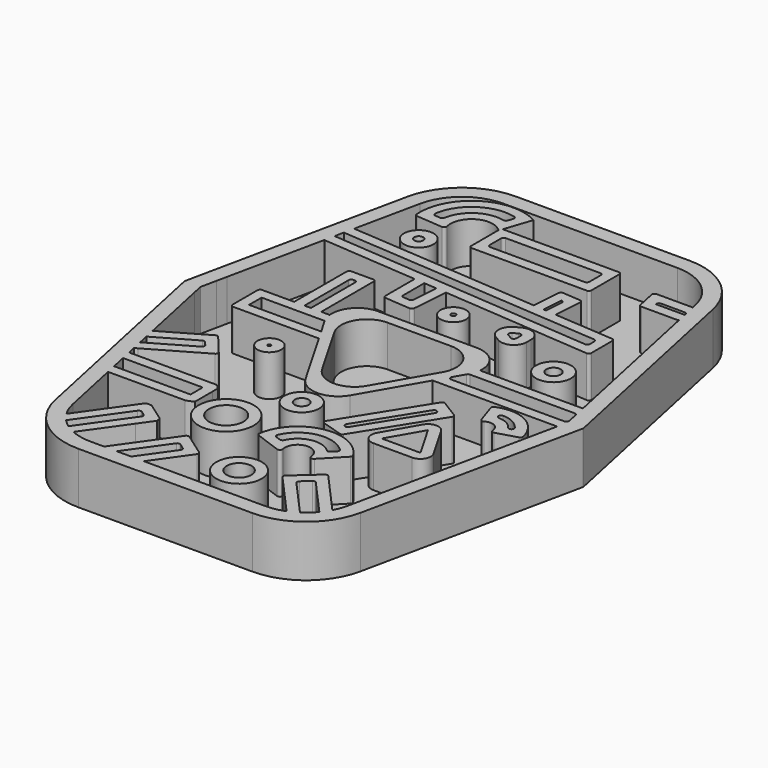
from build123d import *

# Parameters (mm, degrees)
F1_DEPTH = 10
F0_R     = 3.399072215
F0_R_2   = 1.3990718871
F0_R_3   = 2.4667891004
F0_R_4   = 0.4667891482
F0_R_5   = 2.8692483902
F0_R_6   = 0.8692480624
F0_R_7   = 2.3127347231
F0_R_8   = 0.3127347231
F0_R_9   = 4.3970015831
F0_R_10  = 2.39700148
F0_R_11  = 5.3427862003
F0_R_12  = 3.3427864912
F0_R_13  = 3.3629990648
F0_R_14  = 1.3629989638
F2_DEPTH = 2


with BuildPart() as f1:
    # F0 (on Top) → F1 (new body)
    with BuildSketch(Plane.XY):
        with BuildLine():
            ThreePointArc((-38.6444153976, 0.1036928032), (-38.6525607435, 0.0521305146), (-38.6552857598, 0))
            ThreePointArc((-38.6552857598, 0), (-38.6525607435, -0.0521305146), (-38.6444153976, -0.1036928032))
            Line((-38.6444153976, -0.1036928032), (-29.6150769124, -42.6960128826))
            ThreePointArc((-29.6150769124, -42.6960128826), (-25.081587821, -50.1006971906), (-16.8977063297, -53))
            Line((-16.8977063297, -53), (0, -53))
            Line((0, -53), (16.8977063297, -53))
            ThreePointArc((16.8977063297, -53), (25.081587821, -50.1006971906), (29.6150769124, -42.6960128826))
            Line((29.6150769124, -42.6960128826), (38.6444153976, -0.1036928032))
            ThreePointArc((38.6444153976, -0.1036928032), (38.6552857598, 0), (38.6444153976, 0.1036928032))
            Line((38.6444153976, 0.1036928032), (29.6150769124, 42.6960128826))
            ThreePointArc((29.6150769124, 42.6960128826), (25.081587821, 50.1006971906), (16.8977063297, 53))
            Line((16.8977063297, 53), (0, 53))
            Line((0, 53), (-16.8977063297, 53))
            ThreePointArc((-16.8977063297, 53), (-25.081587821, 50.1006971906), (-29.6150769124, 42.6960128826))
            Line((-29.6150769124, 42.6960128826), (-38.6444153976, 0.1036928032))
        make_face()
        with BuildLine():
            Line((-16.8977063297, -40), (-22.671018251, -48.1651007012))
            ThreePointArc((-22.671018251, -48.1651007012), (-23.462448413, -47.5434846975), (-24.1873929575, -46.8454706828))
            Line((-24.1873929575, -46.8454706828), (-17.6647293923, -37.6205741976))
            ThreePointArc((-17.6647293923, -37.6205741976), (-17.3410368605, -37.4164424895), (-16.9678087612, -37.5009847586))
            Line((-16.9678087612, -37.5009847586), (-16.1512996793, -38.078315252))
            ThreePointArc((-16.1512996793, -38.078315252), (-15.9471679712, -38.4020077838), (-16.0317102403, -38.7752358831))
            Line((-16.0317102403, -38.7752358831), (-16.8977063297, -40))
        make_face(mode=Mode.SUBTRACT)
        Polygon((-14.7321429104, -28.4901845949), (-29.5599630094, -28.4901845949), (-30.1859044805, -25.5375541747), (-14.7321429104, -25.5375541747), align=None, mode=Mode.SUBTRACT)
        with BuildLine():
            Line((-9.03667927, -50), (-11.8329823017, -50))
            Line((-11.8329823017, -50), (-6.4127478404, -42.3342509803))
            ThreePointArc((-6.4127478404, -42.3342509803), (-6.0890553086, -42.1301192721), (-5.7158272093, -42.2146615413))
            Line((-5.7158272093, -42.2146615413), (-4.6680736615, -42.9554984604))
            ThreePointArc((-4.6680736615, -42.9554984604), (-4.4639419533, -43.2791909922), (-4.5484842225, -43.6524190915))
            Line((-4.5484842225, -43.6524190915), (-9.03667927, -50))
        make_face(mode=Mode.SUBTRACT)
        with BuildLine():
            Line((-23.2424551979, -15.1969495596), (-31.3818357551, -19.8962231153))
            Line((-31.3818357551, -19.8962231153), (-31.8192990802, -17.8326635315))
            Line((-31.8192990802, -17.8326635315), (-24.3936597276, -13.5454686523))
            ThreePointArc((-24.3936597276, -13.5454686523), (-24.05538108, -13.486336172), (-23.758744916, -13.6593566327))
            Line((-23.758744916, -13.6593566327), (-23.1075403864, -14.4448121362))
            ThreePointArc((-23.1075403864, -14.4448121362), (-23.0003100157, -14.8522155052), (-23.2424551979, -15.1969495596))
        make_face(mode=Mode.SUBTRACT)
        with BuildLine():
            ThreePointArc((24.5828640799, -46.3983083979), (23.5576252344, -47.4595898133), (22.3873711213, -48.3584436635))
            Line((22.3873711213, -48.3584436635), (15.9027415925, -41.1162009459))
            ThreePointArc((15.9027415925, -41.1162009459), (15.7760011816, -40.7551144222), (15.9417089072, -40.4101686886))
            Line((15.9417089072, -40.4101686886), (17.3893763061, -39.1139422117))
            ThreePointArc((17.3893763061, -39.1139422117), (17.7504628298, -38.9872018008), (18.0954085634, -39.1529095263))
            Line((18.0954085634, -39.1529095263), (24.5828640799, -46.3983083979))
        make_face(mode=Mode.SUBTRACT)
        with BuildLine():
            ThreePointArc((-10.4824310448, 1.0520343855), (-10.4824310448, 6.0520343855), (-6.1523040259, 8.5520343855))
            Line((-6.1523040259, 8.5520343855), (6.1523040259, 8.5520343855))
            ThreePointArc((6.1523040259, 8.5520343855), (10.4824310448, 6.0520343855), (10.4824310448, 1.0520343855))
            Line((10.4824310448, 1.0520343855), (9.8750387092, 0))
            Line((9.8750387092, 0), (8.720338116, -2.000000095))
            Line((8.720338116, -2.000000095), (4.3301270189, -9.604068771))
            ThreePointArc((4.3301270189, -9.604068771), (0, -12.104068771), (-4.3301270189, -9.604068771))
            Line((-4.3301270189, -9.604068771), (-8.720338116, -2.000000095))
            Line((-8.720338116, -2.000000095), (-9.8750387092, 0))
            Line((-9.8750387092, 0), (-10.4824310448, 1.0520343855))
        make_face(mode=Mode.SUBTRACT)
        Polygon((-12.1844401645, 0), (-26.1760037392, 0), (-26.1760037392, 3.0520347133), (-13.9465332278, 3.0520347133), align=None, mode=Mode.SUBTRACT)
        with BuildLine():
            Line((-18.213680014, 15.7631627172), (-18.213680014, 5.0520347431))
            Line((-18.213680014, 5.0520347431), (-19.4621123374, 5.0520347431))
            Line((-19.4621123374, 5.0520347431), (-19.4621123374, 15.7631627172))
            ThreePointArc((-19.4621123374, 15.7631627172), (-19.3156657279, 16.1167161078), (-18.9621123374, 16.2631627172))
            Line((-18.9621123374, 16.2631627172), (-18.713680014, 16.2631627172))
            ThreePointArc((-18.713680014, 16.2631627172), (-18.3601266234, 16.1167161078), (-18.213680014, 15.7631627172))
        make_face(mode=Mode.SUBTRACT)
        with BuildLine():
            Line((9.6164062089, 10.5520347133), (-9.6164062089, 10.5520347133))
            ThreePointArc((-9.6164062089, 10.5520347133), (-13.3245054424, 8.9061366907), (-14.5913433974, 5.0520347431))
            Line((-14.5913433974, 5.0520347431), (-16.2136796862, 5.0520347431))
            Line((-16.2136796862, 5.0520347431), (-16.2136796862, 17.763163045))
            ThreePointArc((-16.2136796862, 17.763163045), (-16.3601262956, 18.1167164356), (-16.7136796862, 18.263163045))
            Line((-16.7136796862, 18.263163045), (-20.9621126652, 18.263163045))
            ThreePointArc((-20.9621126652, 18.263163045), (-21.3156660558, 18.1167164356), (-21.4621126652, 17.763163045))
            Line((-21.4621126652, 17.763163045), (-21.4621126652, 5.0520347431))
            Line((-21.4621126652, 5.0520347431), (-27.6760040671, 5.0520347431))
            ThreePointArc((-27.6760040671, 5.0520347431), (-28.0295574577, 4.9055881337), (-28.1760040671, 4.5520347431))
            Line((-28.1760040671, 4.5520347431), (-28.1760040671, 0))
            Line((-28.1760040671, 0), (-28.1760040671, -1.500000095))
            ThreePointArc((-28.1760040671, -1.500000095), (-28.0295574577, -1.8535534856), (-27.6760040671, -2.000000095))
            Line((-27.6760040671, -2.000000095), (-12.1844401645, -2.000000095))
            Line((-12.1844401645, -2.000000095), (-11.0297395713, -2.000000095))
            Line((-11.0297395713, -2.000000095), (-4.3301270189, -13.6040694267))
            ThreePointArc((-4.3301270189, -13.6040694267), (0, -16.1040694267), (4.3301270189, -13.6040694267))
            Line((4.3301270189, -13.6040694267), (11.0297395713, -2.000000095))
            Line((11.0297395713, -2.000000095), (35.1757369785, -2.000000095))
            Line((35.1757369785, -2.000000095), (26.6802990856, -42.0738560635))
            ThreePointArc((26.6802990856, -42.0738560635), (26.297566954, -43.4121284038), (25.7327165891, -44.6842922322))
            Line((25.7327165891, -44.6842922322), (18.2512778003, -36.3287808889))
            ThreePointArc((18.2512778003, -36.3287808889), (17.9063320668, -36.1630731634), (17.545245543, -36.2898135743))
            Line((17.545245543, -36.2898135743), (13.1175802697, -40.2542994517))
            ThreePointArc((13.1175802697, -40.2542994517), (12.9518725442, -40.5992451852), (13.0786129551, -40.960331709))
            Line((13.0786129551, -40.960331709), (20.5530202963, -49.3079901056))
            ThreePointArc((20.5530202963, -49.3079901056), (18.7578271516, -49.8254745701), (16.8977063297, -50))
            Line((16.8977063297, -50), (0, -50))
            Line((0, -50), (-6.5872296722, -50))
            Line((-6.5872296722, -50), (-1.7608013315, -43.1740612727))
            ThreePointArc((-1.7608013315, -43.1740612727), (-1.6762590624, -42.8008331733), (-1.8803907705, -42.4771406415))
            Line((-1.8803907705, -42.4771406415), (-6.1941850281, -39.4269786503))
            ThreePointArc((-6.1941850281, -39.4269786503), (-6.5674131275, -39.3424363812), (-6.8911056593, -39.5465680893))
            Line((-6.8911056593, -39.5465680893), (-13.4660026566, -48.845337464))
            Line((-13.4660026566, -48.845337464), (-14.2824318996, -50))
            Line((-14.2824318996, -50), (-16.8977063297, -50))
            ThreePointArc((-16.8977063297, -50), (-18.9534360088, -49.7864179088), (-20.9213522792, -49.1547950973))
            Line((-20.9213522792, -49.1547950973), (-15.2646851029, -41.1546631526))
            Line((-15.2646851029, -41.1546631526), (-13.3070006372, -38.3859420058))
            ThreePointArc((-13.3070006372, -38.3859420058), (-13.374696737, -37.928816524), (-13.5192652637, -37.4899014877))
            Line((-13.5192652637, -37.4899014877), (-17.0987254889, -34.958966335))
            ThreePointArc((-17.0987254889, -34.958966335), (-17.6772138363, -34.9371997538), (-18.2537530321, -34.9894023189))
            Line((-18.2537530321, -34.9894023189), (-25.4550744561, -45.174113523))
            ThreePointArc((-25.4550744561, -45.174113523), (-26.1977837687, -43.6753992477), (-26.6802990856, -42.0738560635))
            Line((-26.6802990856, -42.0738560635), (-29.1359738983, -30.4901849227))
            Line((-29.1359738983, -30.4901849227), (-14.1564217807, -30.4901849227))
            ThreePointArc((-14.1564217807, -30.4901849227), (-13.4271673617, -30.2402174483), (-12.7321425825, -29.9066963813))
            Line((-12.7321425825, -29.9066963813), (-12.7321425825, -25.6636664271))
            Line((-12.7321425825, -25.6636664271), (-12.7558211848, -24.3296473641))
            ThreePointArc((-12.7558211848, -24.3296473641), (-13.174958101, -23.9125849047), (-13.6320888867, -23.5375538468))
            Line((-13.6320888867, -23.5375538468), (-14.7321429104, -23.5375538468))
            Line((-14.7321429104, -23.5375538468), (-30.6098935916, -23.5375538468))
            Line((-30.6098935916, -23.5375538468), (-30.9456432666, -21.9537880317))
            Line((-30.9456432666, -21.9537880317), (-30.3818358892, -21.6282736906))
            Line((-30.3818358892, -21.6282736906), (-20.1906209234, -15.7443729867))
            ThreePointArc((-20.1906209234, -15.7443729867), (-19.9484757411, -15.3996389323), (-20.0557061118, -14.9922355633))
            Line((-20.0557061118, -14.9922355633), (-23.2966388816, -11.0831588223))
            ThreePointArc((-23.2966388816, -11.0831588223), (-23.5932750456, -10.9101383616), (-23.9315536932, -10.9692708419))
            Line((-23.9315536932, -10.9692708419), (-32.2554915687, -15.7750986151))
            Line((-32.2554915687, -15.7750986151), (-35.1757369785, -2.000000095))
            Line((-35.1757369785, -2.000000095), (-35.5997260402, 0))
            Line((-35.5997260402, 0), (-34.9527114037, 3.0520347133))
            Line((-34.9527114037, 3.0520347133), (-34.5287223558, 5.0520347431))
            Line((-34.5287223558, 5.0520347431), (-30.5607553711, 23.7693438962))
            Line((-30.5607553711, 23.7693438962), (-30.3036586015, 23.7148407898))
            Line((-30.3036586015, 23.7148407898), (-11.898490251, 22.2927000705))
            Line((-11.898490251, 22.2927000705), (-11.898490251, 15.1860698793))
            ThreePointArc((-11.898490251, 15.1860698793), (-11.7654096763, 14.8464080838), (-11.4370097096, 14.6875558361))
            Line((-11.4370097096, 14.6875558361), (-6.4813007835, 14.3046353801))
            ThreePointArc((-6.4813007835, 14.3046353801), (-6.1175160348, 14.4234093925), (-5.9442672817, 14.7646299648))
            Line((-5.9442672817, 14.7646299648), (-5.4013747687, 21.7906773609))
            Line((-5.4013747687, 21.7906773609), (23.6295337142, 19.547501081))
            ThreePointArc((23.6295337142, 19.547501081), (24.0077149683, 19.679095699), (24.1680531728, 20.0460151242))
            Line((24.1680531728, 20.0460151242), (24.1680531728, 25.1655394856))
            ThreePointArc((24.1680531728, 25.1655394856), (24.0340055522, 25.5062429579), (23.7037377487, 25.664264471))
            Line((23.7037377487, 25.664264471), (12.112475713, 26.4936379369))
            Line((12.112475713, 26.4936379369), (12.5044798494, 31.972258669))
            ThreePointArc((12.5044798494, 31.972258669), (12.3836394887, 32.3353622584), (12.0414394399, 32.5066682302))
            Line((12.0414394399, 32.5066682302), (8.5309401818, 32.7578501057))
            ThreePointArc((8.5309401818, 32.7578501057), (8.1678365924, 32.637009745), (7.9965306205, 32.2948096962))
            Line((7.9965306205, 32.2948096962), (7.6045264841, 26.8161889641))
            Line((7.6045264841, 26.8161889641), (-29.3542301857, 29.4606475244))
            Line((-29.3542301857, 29.4606475244), (-26.6802990856, 42.0738560635))
            ThreePointArc((-26.6802990856, 42.0738560635), (-23.1929997846, 47.7697670697), (-16.8977063297, 50))
            Line((-16.8977063297, 50), (0, 50))
            Line((0, 50), (16.8977063297, 50))
            ThreePointArc((16.8977063297, 50), (23.1929997846, 47.7697670697), (26.6802990856, 42.0738560635))
            Line((26.6802990856, 42.0738560635), (26.8416769509, 41.3126200438))
            Line((26.8416769509, 41.3126200438), (19.8224472179, 41.3126200438))
            ThreePointArc((19.8224472179, 41.3126200438), (19.4339588644, 41.1273847165), (19.3333175801, 40.7089272406))
            Line((19.3333175801, 40.7089272406), (20.1082804097, 37.053347716))
            ThreePointArc((20.1082804097, 37.053347716), (20.2826453747, 36.7685521657), (20.5974100474, 36.6570405192))
            Line((20.5974100474, 36.6570405192), (27.4046450229, 36.6570405192))
            Line((27.4046450229, 36.6570405192), (27.8103990355, 36.7430581467))
            Line((27.8103990355, 36.7430581467), (34.5287223558, 5.0520347431))
            Line((34.5287223558, 5.0520347431), (14.5913433974, 5.0520347431))
            ThreePointArc((14.5913433974, 5.0520347431), (13.3245054424, 8.9061366907), (9.6164062089, 10.5520347133))
        make_face(mode=Mode.SUBTRACT)
        with BuildLine():
            Line((-9.8984905148, 17.0374940741), (-9.8984905148, 22.1381629856))
            Line((-9.8984905148, 22.1381629856), (-7.3954306786, 21.9447551749))
            Line((-7.3954306786, 21.9447551749), (-7.7842453776, 16.9127636888))
            ThreePointArc((-7.7842453776, 16.9127636888), (-7.9574941307, 16.5715431165), (-8.3212788794, 16.4527691041))
            Line((-8.3212788794, 16.4527691041), (-9.4370099734, 16.5389800309))
            ThreePointArc((-9.4370099734, 16.5389800309), (-9.7654099401, 16.6978322786), (-9.8984905148, 17.0374940741))
        make_face(mode=Mode.SUBTRACT)
        with BuildLine():
            Line((-30.1495807781, 25.7088968219), (-29.7729517471, 27.4854947711))
            Line((-29.7729517471, 27.4854947711), (21.70373789, 23.8022547265))
            ThreePointArc((21.70373789, 23.8022547265), (22.0340056935, 23.6442332134), (22.1680533141, 23.3035297411))
            Line((22.1680533141, 23.3035297411), (22.1680533141, 22.2065136211))
            ThreePointArc((22.1680533141, 22.2065136211), (22.0077151096, 21.8395941958), (21.6295338555, 21.7079995778))
            Line((21.6295338555, 21.7079995778), (-30.1495807781, 25.7088968219))
        make_face(mode=Mode.SUBTRACT)
        with BuildLine():
            Line((12.6174528664, 0.75), (13.8021956605, 2.8020347133))
            ThreePointArc((13.8021956605, 2.8020347133), (13.9852083624, 2.9850474152), (14.2352083624, 3.0520347133))
            Line((14.2352083624, 3.0520347133), (34.5475967202, 3.0520347133))
            ThreePointArc((34.5475967202, 3.0520347133), (34.8623613929, 2.9405230668), (35.036726358, 2.6557275165))
            Line((35.036726358, 2.6557275165), (35.4717464737, 0.6036928032))
            ThreePointArc((35.4717464737, 0.6036928032), (35.3711051894, 0.1852353273), (34.9826168359, 0))
            Line((34.9826168359, 0), (13.0504655683, 0))
            ThreePointArc((13.0504655683, 0), (12.6174528664, 0.25), (12.6174528664, 0.75))
        make_face(mode=Mode.SUBTRACT)
        with BuildLine():
            Line((10.3668416044, 30.120097031), (10.1175757714, 26.6363762404))
            Line((10.1175757714, 26.6363762404), (9.5994264256, 26.6734506606))
            Line((9.5994264256, 26.6734506606), (9.8843768344, 30.6558964365))
            Line((9.8843768344, 30.6558964365), (9.9038011949, 30.6545065922))
            ThreePointArc((9.9038011949, 30.6545065922), (10.2460012437, 30.4832006204), (10.3668416044, 30.120097031))
        make_face(mode=Mode.SUBTRACT)
        with BuildLine():
            Line((22.2908854137, 39.3126189268), (26.8605515458, 39.3126189268))
            ThreePointArc((26.8605515458, 39.3126189268), (27.1753162185, 39.2011072803), (27.3496811835, 38.91631173))
            Line((27.3496811835, 38.91631173), (27.4046450229, 38.6570416361))
            Line((27.4046450229, 38.6570416361), (21.8127550029, 38.6570416361))
            Line((21.8127550029, 38.6570416361), (21.8017557759, 38.7089261237))
            ThreePointArc((21.8017557759, 38.7089261237), (21.9023970602, 39.1273835996), (22.2908854137, 39.3126189268))
        make_face(mode=Mode.SUBTRACT)
    extrude(amount=F1_DEPTH)


with BuildPart() as f1b:
    # F0 (on Top) → F1, piece 2 (new body)
    with BuildSketch(Plane.XY):
        with BuildLine():
            Line((11.3479569554, 40), (11.3479569554, 42.8686450124))
            ThreePointArc((11.3479569554, 42.8686450124), (11.201510346, 43.222198403), (10.8479569554, 43.3686450124))
            Line((10.8479569554, 43.3686450124), (-11.6518868951, 43.3686450124))
            Line((-11.6518868951, 43.3686450124), (-9.9092187502, 48.610936098))
            ThreePointArc((-9.9092187502, 48.610936098), (-20.2784683686, 48.3517526151), (-24.9408979548, 39.0862108565))
            ThreePointArc((-24.9408979548, 39.0862108565), (-24.7965040915, 38.7701226352), (-24.4809901003, 38.6244782986))
            Line((-24.4809901003, 38.6244782986), (-19.372677463, 38.2275064133))
            ThreePointArc((-19.372677463, 38.2275064133), (-18.9524686823, 38.402768931), (-18.8485632614, 38.8460476615))
            ThreePointArc((-18.8485632614, 38.8460476615), (-16.8871391154, 43.3911768549), (-11.9827720337, 42.7184454137))
            Line((-11.9827720337, 42.7184454137), (-11.9827720337, 36.1013327837))
            ThreePointArc((-11.9827720337, 36.1013327837), (-11.8363254243, 35.7477793931), (-11.4827720337, 35.6013327837))
            Line((-11.4827720337, 35.6013327837), (10.8479569554, 35.6013327837))
            ThreePointArc((10.8479569554, 35.6013327837), (11.201510346, 35.7477793931), (11.3479569554, 36.1013327837))
            Line((11.3479569554, 36.1013327837), (11.3479569554, 40))
        make_face()
        with BuildLine():
            Line((9.3479566276, 40.8686446846), (9.3479566276, 40))
            Line((9.3479566276, 40), (9.3479566276, 38.1013331115))
            ThreePointArc((9.3479566276, 38.1013331115), (9.2015100182, 37.7477797209), (8.8479566276, 37.6013331115))
            Line((8.8479566276, 37.6013331115), (-9.4827717058, 37.6013331115))
            ThreePointArc((-9.4827717058, 37.6013331115), (-9.8363250964, 37.7477797209), (-9.9827717058, 38.1013331115))
            Line((-9.9827717058, 38.1013331115), (-9.9827717058, 40.8686446846))
            ThreePointArc((-9.9827717058, 40.8686446846), (-9.8363250964, 41.2221980751), (-9.4827717058, 41.3686446846))
            Line((-9.4827717058, 41.3686446846), (8.8479566276, 41.3686446846))
            ThreePointArc((8.8479566276, 41.3686446846), (9.2015100182, 41.2221980751), (9.3479566276, 40.8686446846))
        make_face(mode=Mode.SUBTRACT)
        with BuildLine():
            ThreePointArc((-13.4505709735, 45.7493001201), (-18.2466697127, 44.9021356054), (-20.8884646153, 40.8105380538))
            ThreePointArc((-20.8884646153, 40.8105380538), (-21.07314416, 40.4979170999), (-21.4206567051, 40.3926867524))
            Line((-21.4206567051, 40.3926867524), (-22.4207461206, 40.4704046621))
            ThreePointArc((-22.4207461206, 40.4704046621), (-22.77354721, 40.6579409406), (-22.8763290658, 41.0440424228))
            ThreePointArc((-22.8763290658, 41.0440424228), (-19.3529933545, 46.5682854362), (-12.8944386724, 47.6720185674))
            ThreePointArc((-12.8944386724, 47.6720185674), (-12.578470645, 47.4274727229), (-12.5425237403, 47.0295452364))
            Line((-12.5425237403, 47.0295452364), (-12.8589549278, 46.0776575245))
            ThreePointArc((-12.8589549278, 46.0776575245), (-13.0907839452, 45.798205021), (-13.4505709735, 45.7493001201))
        make_face(mode=Mode.SUBTRACT)
    extrude(amount=F1_DEPTH)


with BuildPart() as f1c:
    # F0 (on Top) → F1, piece 3 (new body)
    with BuildSketch(Plane.XY):
        with Locations((23.5671252012, 11.6359107196)):
            Circle(F0_R)
        with Locations((23.5671252012, 11.6359107196)):
            Circle(F0_R_2, mode=Mode.SUBTRACT)
    extrude(amount=F1_DEPTH)


with BuildPart() as f1d:
    # F0 (on Top) → F1, piece 4 (new body)
    with BuildSketch(Plane.XY):
        with BuildLine():
            Line((14.2961637919, 16.6796022979), (14.313119636, 17.6879111175))
            ThreePointArc((14.313119636, 17.6879111175), (13.0996991626, 19.8736857525), (10.6000525651, 19.9157201145))
            Line((10.6000525651, 19.9157201145), (9.7183535904, 19.4262498964))
            ThreePointArc((9.7183535904, 19.4262498964), (8.4321274663, 17.2825096235), (9.6455479397, 15.0967349886))
            Line((9.6455479397, 15.0967349886), (10.5102910703, 14.577896387))
            ThreePointArc((10.5102910703, 14.577896387), (13.0099376678, 14.535862025), (14.2961637919, 16.6796022979))
        make_face()
        with BuildLine():
            ThreePointArc((10.6745288389, 16.8117272069), (10.4318447443, 17.2488821339), (10.6890899691, 17.6776301884))
            Line((10.6890899691, 17.6776301884), (11.5707889438, 18.1671004065))
            ThreePointArc((11.5707889438, 18.1671004065), (12.0707182633, 18.1586935341), (12.313402358, 17.7215386072))
            Line((12.313402358, 17.7215386072), (12.2964465139, 16.7132297875))
            ThreePointArc((12.2964465139, 16.7132297875), (12.0392012891, 16.2844817329), (11.5392719696, 16.2928886053))
            Line((11.5392719696, 16.2928886053), (10.6745288389, 16.8117272069))
        make_face(mode=Mode.SUBTRACT)
    extrude(amount=F1_DEPTH)


with BuildPart() as f1e:
    # F0 (on Top) → F1, piece 5 (new body)
    with BuildSketch(Plane.XY):
        with Locations((0, 16.813468188)):
            Circle(F0_R_3)
        with Locations((0, 16.813468188)):
            Circle(F0_R_4, mode=Mode.SUBTRACT)
    extrude(amount=F1_DEPTH)


with BuildPart() as f1f:
    # F0 (on Top) → F1, piece 6 (new body)
    with BuildSketch(Plane.XY):
        with Locations((-19.6312479675, 32.9623892903)):
            Circle(F0_R_5)
        with Locations((-19.6312479675, 32.9623892903)):
            Circle(F0_R_6, mode=Mode.SUBTRACT)
    extrude(amount=F1_DEPTH)


with BuildPart() as f1g:
    # F0 (on Top) → F1, piece 7 (new body)
    with BuildSketch(Plane.XY):
        with Locations((-15.4942134395, -8.4121655673)):
            Circle(F0_R_7)
        with Locations((-15.4942134395, -8.4121655673)):
            Circle(F0_R_8, mode=Mode.SUBTRACT)
    extrude(amount=F1_DEPTH)


with BuildPart() as f1h:
    # F0 (on Top) → F1, piece 8 (new body)
    with BuildSketch(Plane.XY):
        with BuildLine():
            ThreePointArc((16.9099035396, -29.31134498), (17.0474105448, -29.0174641157), (16.9755778926, -28.7010558209))
            ThreePointArc((16.9755778926, -28.7010558209), (8.0370288338, -24.8624119764), (1.3814706109, -31.9572263209))
            ThreePointArc((1.3814706109, -31.9572263209), (1.4476923266, -32.2852257943), (1.7059395028, -32.4980105827))
            Line((1.7059395028, -32.4980105827), (6.7058357347, -34.3116790255))
            ThreePointArc((6.7058357347, -34.3116790255), (7.2089344656, -34.2149809572), (7.3628591381, -33.7263440321))
            ThreePointArc((7.3628591381, -33.7263440321), (9.3831674608, -30.7137956444), (12.2334222709, -32.9572619412))
            ThreePointArc((12.2334222709, -32.9572619412), (12.5632782348, -33.3877886295), (13.0914250565, -33.2644228284))
            Line((13.0914250565, -33.2644228284), (16.9099035396, -29.31134498))
        make_face()
        with BuildLine():
            ThreePointArc((13.5579327139, -29.9027619507), (13.2087280029, -30.0552754711), (12.8534722744, -29.9174434304))
            ThreePointArc((12.8534722744, -29.9174434304), (8.9077745167, -28.7672002682), (5.6891479067, -31.3229844675))
            ThreePointArc((5.6891479067, -31.3229844675), (5.4279014723, -31.5785333578), (5.062574615, -31.5880843862))
            Line((5.062574615, -31.5880843862), (4.120345984, -31.2462992261))
            ThreePointArc((4.120345984, -31.2462992261), (3.8315880544, -30.9739599037), (3.832254111, -30.5770349678))
            ThreePointArc((3.832254111, -30.5770349678), (8.4869300114, -26.8117435782), (14.2383441665, -28.4744709171))
            ThreePointArc((14.2383441665, -28.4744709171), (14.3929775253, -28.8260001172), (14.2527028416, -29.18350154))
            Line((14.2527028416, -29.18350154), (13.5579327139, -29.9027619507))
        make_face(mode=Mode.SUBTRACT)
    extrude(amount=F1_DEPTH)


with BuildPart() as f1i:
    # F0 (on Top) → F1, piece 9 (new body)
    with BuildSketch(Plane.XY):
        with BuildLine():
            ThreePointArc((10.9588627462, -24.4177700551), (11.2812815043, -24.4095095453), (11.5315792264, -24.2061056565))
            Line((11.5315792264, -24.2061056565), (20.7565783394, -9.4918535856))
            ThreePointArc((20.7565783394, -9.4918535856), (20.820301645, -9.1145129574), (20.5985407094, -8.8026336588))
            Line((20.5985407094, -8.8026336588), (17.1937893426, -6.6680482115))
            ThreePointArc((17.1937893426, -6.6680482115), (16.8164487143, -6.604324906), (16.5045694158, -6.8260858415))
            Line((16.5045694158, -6.8260858415), (6.7180857243, -22.4359288517))
            ThreePointArc((6.7180857243, -22.4359288517), (6.6727194656, -22.8748510565), (6.992626801, -23.1787755471))
            Line((6.992626801, -23.1787755471), (10.9588627462, -24.4177700551))
        make_face()
        with BuildLine():
            Line((17.9996980174, -10.1240042467), (10.6561208163, -21.8373111766))
            ThreePointArc((10.6561208163, -21.8373111766), (10.4058230943, -22.0407150654), (10.0834043362, -22.0489755752))
            Line((10.0834043362, -22.0489755752), (10.0650914715, -22.0432549023))
            ThreePointArc((10.0650914715, -22.0432549023), (9.7451841361, -21.7393304116), (9.7905503948, -21.3004082068))
            Line((9.7905503948, -21.3004082068), (17.1367200769, -9.5829661635))
            ThreePointArc((17.1367200769, -9.5829661635), (17.4485993754, -9.361205228), (17.8259400037, -9.4249285335))
            Line((17.8259400037, -9.4249285335), (17.8416603874, -9.4347843199))
            ThreePointArc((17.8416603874, -9.4347843199), (18.063421323, -9.7466636185), (17.9996980174, -10.1240042467))
        make_face(mode=Mode.SUBTRACT)
    extrude(amount=F1_DEPTH)


with BuildPart() as f1j:
    # F0 (on Top) → F1, piece 10 (new body)
    with BuildSketch(Plane.XY):
        with BuildLine():
            Line((18.923042907, -14.1690840721), (15.1665538036, -20.6755140573))
            ThreePointArc((15.1665538036, -20.6755140573), (15.1665538036, -22.6755140573), (16.8986046112, -23.6755140573))
            Line((16.8986046112, -23.6755140573), (24.411582818, -23.6755140573))
            ThreePointArc((24.411582818, -23.6755140573), (26.1436336256, -22.6755140573), (26.1436336256, -20.6755140573))
            Line((26.1436336256, -20.6755140573), (22.3871445222, -14.1690840721))
            ThreePointArc((22.3871445222, -14.1690840721), (20.6550937146, -13.1690840721), (18.923042907, -14.1690840721))
        make_face()
        Polygon((20.6550937146, -15.1690840721), (24.411582818, -21.6755140573), (16.8986046112, -21.6755140573), align=None, mode=Mode.SUBTRACT)
    extrude(amount=F1_DEPTH)


with BuildPart() as f1k:
    # F0 (on Top) → F1, piece 11 (new body)
    with BuildSketch(Plane.XY):
        with BuildLine():
            ThreePointArc((32.8763900957, -8.4079776533), (33.1630589547, -8.1865017518), (33.2249246203, -7.8295658344))
            ThreePointArc((33.2249246203, -7.8295658344), (29.6755894977, -3.1174797736), (23.7793687223, -2.9274391838))
            ThreePointArc((23.7793687223, -2.9274391838), (23.5231046031, -3.1834847089), (23.5070086443, -3.545384598))
            Line((23.5070086443, -3.545384598), (24.8027076737, -7.3750600447))
            ThreePointArc((24.8027076737, -7.3750600447), (25.1102601617, -7.686430869), (25.5450522942, -7.6364696377))
            ThreePointArc((25.5450522942, -7.6364696377), (27.3723630932, -7.5554013738), (28.3578934548, -9.0962993995))
            ThreePointArc((28.3578934548, -9.0962993995), (28.5673105079, -9.480597228), (28.9989564669, -9.5528612523))
            Line((28.9989564669, -9.5528612523), (32.8763900957, -8.4079776533))
        make_face()
        with BuildLine():
            ThreePointArc((30.1779519109, -7.119379395), (29.875095979, -7.1131259252), (29.6314312689, -6.9331583438))
            ThreePointArc((29.6314312689, -6.9331583438), (28.293653655, -5.7802327337), (26.580839153, -5.3499387776))
            ThreePointArc((26.580839153, -5.3499387776), (26.2934192175, -5.2542799985), (26.1139781478, -5.0102272914))
            ThreePointArc((26.1139781478, -5.0102272914), (26.1833094189, -4.5557989091), (26.5943705728, -4.3500303314))
            ThreePointArc((26.5943705728, -4.3500303314), (28.7542989359, -4.8926484136), (30.4412906145, -6.346534239))
            ThreePointArc((30.4412906145, -6.346534239), (30.5096405755, -6.801111254), (30.1779519109, -7.119379395))
        make_face(mode=Mode.SUBTRACT)
    extrude(amount=F1_DEPTH)


with BuildPart() as f1l:
    # F0 (on Top) → F1, piece 12 (new body)
    with BuildSketch(Plane.XY):
        with Locations((6.5540773794, -43.3322489262)):
            Circle(F0_R_9)
        with Locations((6.5540773794, -43.3322489262)):
            Circle(F0_R_10, mode=Mode.SUBTRACT)
    extrude(amount=F1_DEPTH)


with BuildPart() as f1m:
    # F0 (on Top) → F1, piece 13 (new body)
    with BuildSketch(Plane.XY):
        with Locations((-6.242133677, -30.4548274726)):
            Circle(F0_R_11)
        with Locations((-6.242133677, -30.4548274726)):
            Circle(F0_R_12, mode=Mode.SUBTRACT)
    extrude(amount=F1_DEPTH)


with BuildPart() as f1n:
    # F0 (on Top) → F1, piece 14 (new body)
    with BuildSketch(Plane.XY):
        with Locations((0, -19.9465807527)):
            Circle(F0_R_13)
        with Locations((0, -19.9465807527)):
            Circle(F0_R_14, mode=Mode.SUBTRACT)
    extrude(amount=F1_DEPTH)


with BuildPart() as f2:
    # F0 (on Top) → F2 (new body)
    with BuildSketch(Plane.XY):
        with BuildLine():
            ThreePointArc((-14.5913433974, 5.0520347431), (-13.3245054424, 8.9061366907), (-9.6164062089, 10.5520347133))
            Line((-9.6164062089, 10.5520347133), (9.6164062089, 10.5520347133))
            ThreePointArc((9.6164062089, 10.5520347133), (13.3245054424, 8.9061366907), (14.5913433974, 5.0520347431))
            Line((14.5913433974, 5.0520347431), (34.5287223558, 5.0520347431))
            Line((34.5287223558, 5.0520347431), (27.8103990355, 36.7430581467))
            Line((27.8103990355, 36.7430581467), (27.4046450229, 36.6570405192))
            Line((27.4046450229, 36.6570405192), (20.5974100474, 36.6570405192))
            ThreePointArc((20.5974100474, 36.6570405192), (20.2826453747, 36.7685521657), (20.1082804097, 37.053347716))
            Line((20.1082804097, 37.053347716), (19.3333175801, 40.7089272406))
            ThreePointArc((19.3333175801, 40.7089272406), (19.4339588644, 41.1273847165), (19.8224472179, 41.3126200438))
            Line((19.8224472179, 41.3126200438), (26.8416769509, 41.3126200438))
            Line((26.8416769509, 41.3126200438), (26.6802990856, 42.0738560635))
            ThreePointArc((26.6802990856, 42.0738560635), (23.1929997846, 47.7697670697), (16.8977063297, 50))
            Line((16.8977063297, 50), (0, 50))
            Line((0, 50), (-16.8977063297, 50))
            ThreePointArc((-16.8977063297, 50), (-23.1929997846, 47.7697670697), (-26.6802990856, 42.0738560635))
            Line((-26.6802990856, 42.0738560635), (-29.3542301857, 29.4606475244))
            Line((-29.3542301857, 29.4606475244), (7.6045264841, 26.8161889641))
            Line((7.6045264841, 26.8161889641), (7.9965306205, 32.2948096962))
            ThreePointArc((7.9965306205, 32.2948096962), (8.1678365924, 32.637009745), (8.5309401818, 32.7578501057))
            Line((8.5309401818, 32.7578501057), (12.0414394399, 32.5066682302))
            ThreePointArc((12.0414394399, 32.5066682302), (12.3836394887, 32.3353622584), (12.5044798494, 31.972258669))
            Line((12.5044798494, 31.972258669), (12.112475713, 26.4936379369))
            Line((12.112475713, 26.4936379369), (23.7037377487, 25.664264471))
            ThreePointArc((23.7037377487, 25.664264471), (24.0340055522, 25.5062429579), (24.1680531728, 25.1655394856))
            Line((24.1680531728, 25.1655394856), (24.1680531728, 20.0460151242))
            ThreePointArc((24.1680531728, 20.0460151242), (24.0077149683, 19.679095699), (23.6295337142, 19.547501081))
            Line((23.6295337142, 19.547501081), (-5.4013747687, 21.7906773609))
            Line((-5.4013747687, 21.7906773609), (-5.9442672817, 14.7646299648))
            ThreePointArc((-5.9442672817, 14.7646299648), (-6.1175160348, 14.4234093925), (-6.4813007835, 14.3046353801))
            Line((-6.4813007835, 14.3046353801), (-11.4370097096, 14.6875558361))
            ThreePointArc((-11.4370097096, 14.6875558361), (-11.7654096763, 14.8464080838), (-11.898490251, 15.1860698793))
            Line((-11.898490251, 15.1860698793), (-11.898490251, 22.2927000705))
            Line((-11.898490251, 22.2927000705), (-30.3036586015, 23.7148407898))
            Line((-30.3036586015, 23.7148407898), (-30.5607553711, 23.7693438962))
            Line((-30.5607553711, 23.7693438962), (-34.5287223558, 5.0520347431))
            Line((-34.5287223558, 5.0520347431), (-34.9527114037, 3.0520347133))
            Line((-34.9527114037, 3.0520347133), (-35.5997260402, 0))
            Line((-35.5997260402, 0), (-35.1757369785, -2.000000095))
            Line((-35.1757369785, -2.000000095), (-32.2554915687, -15.7750986151))
            Line((-32.2554915687, -15.7750986151), (-23.9315536932, -10.9692708419))
            ThreePointArc((-23.9315536932, -10.9692708419), (-23.5932750456, -10.9101383616), (-23.2966388816, -11.0831588223))
            Line((-23.2966388816, -11.0831588223), (-20.0557061118, -14.9922355633))
            ThreePointArc((-20.0557061118, -14.9922355633), (-19.9484757411, -15.3996389323), (-20.1906209234, -15.7443729867))
            Line((-20.1906209234, -15.7443729867), (-30.3818358892, -21.6282736906))
            Line((-30.3818358892, -21.6282736906), (-30.9456432666, -21.9537880317))
            Line((-30.9456432666, -21.9537880317), (-30.6098935916, -23.5375538468))
            Line((-30.6098935916, -23.5375538468), (-14.7321429104, -23.5375538468))
            Line((-14.7321429104, -23.5375538468), (-13.6320888867, -23.5375538468))
            ThreePointArc((-13.6320888867, -23.5375538468), (-13.174958101, -23.9125849047), (-12.7558211848, -24.3296473641))
            Line((-12.7558211848, -24.3296473641), (-12.7321425825, -25.6636664271))
            Line((-12.7321425825, -25.6636664271), (-12.7321425825, -29.9066963813))
            ThreePointArc((-12.7321425825, -29.9066963813), (-13.4271673617, -30.2402174483), (-14.1564217807, -30.4901849227))
            Line((-14.1564217807, -30.4901849227), (-29.1359738983, -30.4901849227))
            Line((-29.1359738983, -30.4901849227), (-26.6802990856, -42.0738560635))
            ThreePointArc((-26.6802990856, -42.0738560635), (-26.1977837687, -43.6753992477), (-25.4550744561, -45.174113523))
            Line((-25.4550744561, -45.174113523), (-18.2537530321, -34.9894023189))
            ThreePointArc((-18.2537530321, -34.9894023189), (-17.6772138363, -34.9371997538), (-17.0987254889, -34.958966335))
            Line((-17.0987254889, -34.958966335), (-13.5192652637, -37.4899014877))
            ThreePointArc((-13.5192652637, -37.4899014877), (-13.374696737, -37.928816524), (-13.3070006372, -38.3859420058))
            Line((-13.3070006372, -38.3859420058), (-15.2646851029, -41.1546631526))
            Line((-15.2646851029, -41.1546631526), (-20.9213522792, -49.1547950973))
            ThreePointArc((-20.9213522792, -49.1547950973), (-18.9534360088, -49.7864179088), (-16.8977063297, -50))
            Line((-16.8977063297, -50), (-14.2824318996, -50))
            Line((-14.2824318996, -50), (-13.4660026566, -48.845337464))
            Line((-13.4660026566, -48.845337464), (-6.8911056593, -39.5465680893))
            ThreePointArc((-6.8911056593, -39.5465680893), (-6.5674131275, -39.3424363812), (-6.1941850281, -39.4269786503))
            Line((-6.1941850281, -39.4269786503), (-1.8803907705, -42.4771406415))
            ThreePointArc((-1.8803907705, -42.4771406415), (-1.6762590624, -42.8008331733), (-1.7608013315, -43.1740612727))
            Line((-1.7608013315, -43.1740612727), (-6.5872296722, -50))
            Line((-6.5872296722, -50), (0, -50))
            Line((0, -50), (16.8977063297, -50))
            ThreePointArc((16.8977063297, -50), (18.7578271516, -49.8254745701), (20.5530202963, -49.3079901056))
            Line((20.5530202963, -49.3079901056), (13.0786129551, -40.960331709))
            ThreePointArc((13.0786129551, -40.960331709), (12.9518725442, -40.5992451852), (13.1175802697, -40.2542994517))
            Line((13.1175802697, -40.2542994517), (17.545245543, -36.2898135743))
            ThreePointArc((17.545245543, -36.2898135743), (17.9063320668, -36.1630731634), (18.2512778003, -36.3287808889))
            Line((18.2512778003, -36.3287808889), (25.7327165891, -44.6842922322))
            ThreePointArc((25.7327165891, -44.6842922322), (26.297566954, -43.4121284038), (26.6802990856, -42.0738560635))
            Line((26.6802990856, -42.0738560635), (35.1757369785, -2.000000095))
            Line((35.1757369785, -2.000000095), (11.0297395713, -2.000000095))
            Line((11.0297395713, -2.000000095), (4.3301270189, -13.6040694267))
            ThreePointArc((4.3301270189, -13.6040694267), (0, -16.1040694267), (-4.3301270189, -13.6040694267))
            Line((-4.3301270189, -13.6040694267), (-11.0297395713, -2.000000095))
            Line((-11.0297395713, -2.000000095), (-12.1844401645, -2.000000095))
            Line((-12.1844401645, -2.000000095), (-27.6760040671, -2.000000095))
            ThreePointArc((-27.6760040671, -2.000000095), (-28.0295574577, -1.8535534856), (-28.1760040671, -1.500000095))
            Line((-28.1760040671, -1.500000095), (-28.1760040671, 0))
            Line((-28.1760040671, 0), (-28.1760040671, 4.5520347431))
            ThreePointArc((-28.1760040671, 4.5520347431), (-28.0295574577, 4.9055881337), (-27.6760040671, 5.0520347431))
            Line((-27.6760040671, 5.0520347431), (-21.4621126652, 5.0520347431))
            Line((-21.4621126652, 5.0520347431), (-21.4621126652, 17.763163045))
            ThreePointArc((-21.4621126652, 17.763163045), (-21.3156660558, 18.1167164356), (-20.9621126652, 18.263163045))
            Line((-20.9621126652, 18.263163045), (-16.7136796862, 18.263163045))
            ThreePointArc((-16.7136796862, 18.263163045), (-16.3601262956, 18.1167164356), (-16.2136796862, 17.763163045))
            Line((-16.2136796862, 17.763163045), (-16.2136796862, 5.0520347431))
            Line((-16.2136796862, 5.0520347431), (-14.5913433974, 5.0520347431))
        make_face()
        with Locations((-6.242133677, -30.4548274726)):
            Circle(F0_R_11, mode=Mode.SUBTRACT)
        with Locations((-15.4942134395, -8.4121655673)):
            Circle(F0_R_7, mode=Mode.SUBTRACT)
        with Locations((6.5540773794, -43.3322489262)):
            Circle(F0_R_9, mode=Mode.SUBTRACT)
        with BuildLine():
            ThreePointArc((1.3814706109, -31.9572263209), (8.0370288338, -24.8624119764), (16.9755778926, -28.7010558209))
            ThreePointArc((16.9755778926, -28.7010558209), (17.0474105448, -29.0174641157), (16.9099035396, -29.31134498))
            Line((16.9099035396, -29.31134498), (13.0914250565, -33.2644228284))
            ThreePointArc((13.0914250565, -33.2644228284), (12.5632782348, -33.3877886295), (12.2334222709, -32.9572619412))
            ThreePointArc((12.2334222709, -32.9572619412), (9.3831674608, -30.7137956444), (7.3628591381, -33.7263440321))
            ThreePointArc((7.3628591381, -33.7263440321), (7.2089344656, -34.2149809572), (6.7058357347, -34.3116790255))
            Line((6.7058357347, -34.3116790255), (1.7059395028, -32.4980105827))
            ThreePointArc((1.7059395028, -32.4980105827), (1.4476923266, -32.2852257943), (1.3814706109, -31.9572263209))
        make_face(mode=Mode.SUBTRACT)
        with Locations((0, -19.9465807527)):
            Circle(F0_R_13, mode=Mode.SUBTRACT)
        with BuildLine():
            Line((20.7565783394, -9.4918535856), (11.5315792264, -24.2061056565))
            ThreePointArc((11.5315792264, -24.2061056565), (11.2812815043, -24.4095095453), (10.9588627462, -24.4177700551))
            Line((10.9588627462, -24.4177700551), (6.992626801, -23.1787755471))
            ThreePointArc((6.992626801, -23.1787755471), (6.6727194656, -22.8748510565), (6.7180857243, -22.4359288517))
            Line((6.7180857243, -22.4359288517), (16.5045694158, -6.8260858415))
            ThreePointArc((16.5045694158, -6.8260858415), (16.8164487143, -6.604324906), (17.1937893426, -6.6680482115))
            Line((17.1937893426, -6.6680482115), (20.5985407094, -8.8026336588))
            ThreePointArc((20.5985407094, -8.8026336588), (20.820301645, -9.1145129574), (20.7565783394, -9.4918535856))
        make_face(mode=Mode.SUBTRACT)
        with BuildLine():
            ThreePointArc((16.8986046112, -23.6755140573), (15.1665538036, -22.6755140573), (15.1665538036, -20.6755140573))
            Line((15.1665538036, -20.6755140573), (18.923042907, -14.1690840721))
            ThreePointArc((18.923042907, -14.1690840721), (20.6550937146, -13.1690840721), (22.3871445222, -14.1690840721))
            Line((22.3871445222, -14.1690840721), (26.1436336256, -20.6755140573))
            ThreePointArc((26.1436336256, -20.6755140573), (26.1436336256, -22.6755140573), (24.411582818, -23.6755140573))
            Line((24.411582818, -23.6755140573), (16.8986046112, -23.6755140573))
        make_face(mode=Mode.SUBTRACT)
        with BuildLine():
            ThreePointArc((23.7793687223, -2.9274391838), (29.6755894977, -3.1174797736), (33.2249246203, -7.8295658344))
            ThreePointArc((33.2249246203, -7.8295658344), (33.1630589547, -8.1865017518), (32.8763900957, -8.4079776533))
            Line((32.8763900957, -8.4079776533), (28.9989564669, -9.5528612523))
            ThreePointArc((28.9989564669, -9.5528612523), (28.5673105079, -9.480597228), (28.3578934548, -9.0962993995))
            ThreePointArc((28.3578934548, -9.0962993995), (27.3723630932, -7.5554013738), (25.5450522942, -7.6364696377))
            ThreePointArc((25.5450522942, -7.6364696377), (25.1102601617, -7.686430869), (24.8027076737, -7.3750600447))
            Line((24.8027076737, -7.3750600447), (23.5070086443, -3.545384598))
            ThreePointArc((23.5070086443, -3.545384598), (23.5231046031, -3.1834847089), (23.7793687223, -2.9274391838))
        make_face(mode=Mode.SUBTRACT)
        with Locations((-19.6312479675, 32.9623892903)):
            Circle(F0_R_5, mode=Mode.SUBTRACT)
        with BuildLine():
            ThreePointArc((10.8479569554, 43.3686450124), (11.201510346, 43.222198403), (11.3479569554, 42.8686450124))
            Line((11.3479569554, 42.8686450124), (11.3479569554, 40))
            Line((11.3479569554, 40), (11.3479569554, 36.1013327837))
            ThreePointArc((11.3479569554, 36.1013327837), (11.201510346, 35.7477793931), (10.8479569554, 35.6013327837))
            Line((10.8479569554, 35.6013327837), (-11.4827720337, 35.6013327837))
            ThreePointArc((-11.4827720337, 35.6013327837), (-11.8363254243, 35.7477793931), (-11.9827720337, 36.1013327837))
            Line((-11.9827720337, 36.1013327837), (-11.9827720337, 42.7184454137))
            ThreePointArc((-11.9827720337, 42.7184454137), (-16.8871391154, 43.3911768549), (-18.8485632614, 38.8460476615))
            ThreePointArc((-18.8485632614, 38.8460476615), (-18.9524686823, 38.402768931), (-19.372677463, 38.2275064133))
            Line((-19.372677463, 38.2275064133), (-24.4809901003, 38.6244782986))
            ThreePointArc((-24.4809901003, 38.6244782986), (-24.7965040915, 38.7701226352), (-24.9408979548, 39.0862108565))
            ThreePointArc((-24.9408979548, 39.0862108565), (-20.2784683686, 48.3517526151), (-9.9092187502, 48.610936098))
            Line((-9.9092187502, 48.610936098), (-11.6518868951, 43.3686450124))
            Line((-11.6518868951, 43.3686450124), (10.8479569554, 43.3686450124))
        make_face(mode=Mode.SUBTRACT)
        with Locations((0, 16.813468188)):
            Circle(F0_R_3, mode=Mode.SUBTRACT)
        with BuildLine():
            ThreePointArc((10.6000525651, 19.9157201145), (13.0996991626, 19.8736857525), (14.313119636, 17.6879111175))
            Line((14.313119636, 17.6879111175), (14.2961637919, 16.6796022979))
            ThreePointArc((14.2961637919, 16.6796022979), (13.0099376678, 14.535862025), (10.5102910703, 14.577896387))
            Line((10.5102910703, 14.577896387), (9.6455479397, 15.0967349886))
            ThreePointArc((9.6455479397, 15.0967349886), (8.4321274663, 17.2825096235), (9.7183535904, 19.4262498964))
            Line((9.7183535904, 19.4262498964), (10.6000525651, 19.9157201145))
        make_face(mode=Mode.SUBTRACT)
        with Locations((23.5671252012, 11.6359107196)):
            Circle(F0_R, mode=Mode.SUBTRACT)
    extrude(amount=F2_DEPTH)


with BuildPart() as f2b:
    # F0 (on Top) → F2, piece 2 (new body)
    with BuildSketch(Plane.XY):
        with BuildLine():
            Line((-19.4621123374, 5.0520347431), (-18.213680014, 5.0520347431))
            Line((-18.213680014, 5.0520347431), (-18.213680014, 15.7631627172))
            ThreePointArc((-18.213680014, 15.7631627172), (-18.3601266234, 16.1167161078), (-18.713680014, 16.2631627172))
            Line((-18.713680014, 16.2631627172), (-18.9621123374, 16.2631627172))
            ThreePointArc((-18.9621123374, 16.2631627172), (-19.3156657279, 16.1167161078), (-19.4621123374, 15.7631627172))
            Line((-19.4621123374, 15.7631627172), (-19.4621123374, 5.0520347431))
        make_face()
    extrude(amount=F2_DEPTH)


with BuildPart() as f2c:
    # F0 (on Top) → F2, piece 3 (new body)
    with BuildSketch(Plane.XY):
        Polygon((-26.1760037392, 3.0520347133), (-26.1760037392, 0), (-12.1844401645, 0), (-13.9465332278, 3.0520347133), align=None)
    extrude(amount=F2_DEPTH)


with BuildPart() as f2d:
    # F0 (on Top) → F2, piece 4 (new body)
    with BuildSketch(Plane.XY):
        with BuildLine():
            Line((6.1523040259, 8.5520343855), (-6.1523040259, 8.5520343855))
            ThreePointArc((-6.1523040259, 8.5520343855), (-10.4824310448, 6.0520343855), (-10.4824310448, 1.0520343855))
            Line((-10.4824310448, 1.0520343855), (-9.8750387092, 0))
            Line((-9.8750387092, 0), (-8.720338116, -2.000000095))
            Line((-8.720338116, -2.000000095), (-4.3301270189, -9.604068771))
            ThreePointArc((-4.3301270189, -9.604068771), (0, -12.104068771), (4.3301270189, -9.604068771))
            Line((4.3301270189, -9.604068771), (8.720338116, -2.000000095))
            Line((8.720338116, -2.000000095), (9.8750387092, 0))
            Line((9.8750387092, 0), (10.4824310448, 1.0520343855))
            ThreePointArc((10.4824310448, 1.0520343855), (10.4824310448, 6.0520343855), (6.1523040259, 8.5520343855))
        make_face()
    extrude(amount=F2_DEPTH)


with BuildPart() as f2e:
    # F0 (on Top) → F2, piece 5 (new body)
    with BuildSketch(Plane.XY):
        with BuildLine():
            ThreePointArc((14.2352083624, 3.0520347133), (13.9852083624, 2.9850474152), (13.8021956605, 2.8020347133))
            Line((13.8021956605, 2.8020347133), (12.6174528664, 0.75))
            ThreePointArc((12.6174528664, 0.75), (12.6174528664, 0.25), (13.0504655683, 0))
            Line((13.0504655683, 0), (34.9826168359, 0))
            ThreePointArc((34.9826168359, 0), (35.3711051894, 0.1852353273), (35.4717464737, 0.6036928032))
            Line((35.4717464737, 0.6036928032), (35.036726358, 2.6557275165))
            ThreePointArc((35.036726358, 2.6557275165), (34.8623613929, 2.9405230668), (34.5475967202, 3.0520347133))
            Line((34.5475967202, 3.0520347133), (14.2352083624, 3.0520347133))
        make_face()
    extrude(amount=F2_DEPTH)


with BuildPart() as f2f:
    # F0 (on Top) → F2, piece 6 (new body)
    with BuildSketch(Plane.XY):
        with BuildLine():
            ThreePointArc((26.580839153, -5.3499387776), (28.293653655, -5.7802327337), (29.6314312689, -6.9331583438))
            ThreePointArc((29.6314312689, -6.9331583438), (29.875095979, -7.1131259252), (30.1779519109, -7.119379395))
            ThreePointArc((30.1779519109, -7.119379395), (30.5096405755, -6.801111254), (30.4412906145, -6.346534239))
            ThreePointArc((30.4412906145, -6.346534239), (28.7542989359, -4.8926484136), (26.5943705728, -4.3500303314))
            ThreePointArc((26.5943705728, -4.3500303314), (26.1833094189, -4.5557989091), (26.1139781478, -5.0102272914))
            ThreePointArc((26.1139781478, -5.0102272914), (26.2934192175, -5.2542799985), (26.580839153, -5.3499387776))
        make_face()
    extrude(amount=F2_DEPTH)


with BuildPart() as f2g:
    # F0 (on Top) → F2, piece 7 (new body)
    with BuildSketch(Plane.XY):
        with BuildLine():
            ThreePointArc((10.0834043362, -22.0489755752), (10.4058230943, -22.0407150654), (10.6561208163, -21.8373111766))
            Line((10.6561208163, -21.8373111766), (17.9996980174, -10.1240042467))
            ThreePointArc((17.9996980174, -10.1240042467), (18.063421323, -9.7466636185), (17.8416603874, -9.4347843199))
            Line((17.8416603874, -9.4347843199), (17.8259400037, -9.4249285335))
            ThreePointArc((17.8259400037, -9.4249285335), (17.4485993754, -9.361205228), (17.1367200769, -9.5829661635))
            Line((17.1367200769, -9.5829661635), (9.7905503948, -21.3004082068))
            ThreePointArc((9.7905503948, -21.3004082068), (9.7451841361, -21.7393304116), (10.0650914715, -22.0432549023))
            Line((10.0650914715, -22.0432549023), (10.0834043362, -22.0489755752))
        make_face()
    extrude(amount=F2_DEPTH)


with BuildPart() as f2h:
    # F0 (on Top) → F2, piece 8 (new body)
    with BuildSketch(Plane.XY):
        Polygon((16.8986046112, -21.6755140573), (24.411582818, -21.6755140573), (20.6550937146, -15.1690840721), align=None)
    extrude(amount=F2_DEPTH)


with BuildPart() as f2i:
    # F0 (on Top) → F2, piece 9 (new body)
    with BuildSketch(Plane.XY):
        with BuildLine():
            ThreePointArc((5.6891479067, -31.3229844675), (8.9077745167, -28.7672002682), (12.8534722744, -29.9174434304))
            ThreePointArc((12.8534722744, -29.9174434304), (13.2087280029, -30.0552754711), (13.5579327139, -29.9027619507))
            Line((13.5579327139, -29.9027619507), (14.2527028416, -29.18350154))
            ThreePointArc((14.2527028416, -29.18350154), (14.3929775253, -28.8260001172), (14.2383441665, -28.4744709171))
            ThreePointArc((14.2383441665, -28.4744709171), (8.4869300114, -26.8117435782), (3.832254111, -30.5770349678))
            ThreePointArc((3.832254111, -30.5770349678), (3.8315880544, -30.9739599037), (4.120345984, -31.2462992261))
            Line((4.120345984, -31.2462992261), (5.062574615, -31.5880843862))
            ThreePointArc((5.062574615, -31.5880843862), (5.4279014723, -31.5785333578), (5.6891479067, -31.3229844675))
        make_face()
    extrude(amount=F2_DEPTH)


with BuildPart() as f2j:
    # F0 (on Top) → F2, piece 10 (new body)
    with BuildSketch(Plane.XY):
        with Locations((0, -19.9465807527)):
            Circle(F0_R_14)
    extrude(amount=F2_DEPTH)


with BuildPart() as f2k:
    # F0 (on Top) → F2, piece 11 (new body)
    with BuildSketch(Plane.XY):
        with BuildLine():
            Line((-7.3954306786, 21.9447551749), (-9.8984905148, 22.1381629856))
            Line((-9.8984905148, 22.1381629856), (-9.8984905148, 17.0374940741))
            ThreePointArc((-9.8984905148, 17.0374940741), (-9.7654099401, 16.6978322786), (-9.4370099734, 16.5389800309))
            Line((-9.4370099734, 16.5389800309), (-8.3212788794, 16.4527691041))
            ThreePointArc((-8.3212788794, 16.4527691041), (-7.9574941307, 16.5715431165), (-7.7842453776, 16.9127636888))
            Line((-7.7842453776, 16.9127636888), (-7.3954306786, 21.9447551749))
        make_face()
    extrude(amount=F2_DEPTH)


with BuildPart() as f2l:
    # F0 (on Top) → F2, piece 12 (new body)
    with BuildSketch(Plane.XY):
        with BuildLine():
            Line((21.70373789, 23.8022547265), (-29.7729517471, 27.4854947711))
            Line((-29.7729517471, 27.4854947711), (-30.1495807781, 25.7088968219))
            Line((-30.1495807781, 25.7088968219), (21.6295338555, 21.7079995778))
            ThreePointArc((21.6295338555, 21.7079995778), (22.0077151096, 21.8395941958), (22.1680533141, 22.2065136211))
            Line((22.1680533141, 22.2065136211), (22.1680533141, 23.3035297411))
            ThreePointArc((22.1680533141, 23.3035297411), (22.0340056935, 23.6442332134), (21.70373789, 23.8022547265))
        make_face()
    extrude(amount=F2_DEPTH)


with BuildPart() as f2m:
    # F0 (on Top) → F2, piece 13 (new body)
    with BuildSketch(Plane.XY):
        with BuildLine():
            Line((9.5994264256, 26.6734506606), (10.1175757714, 26.6363762404))
            Line((10.1175757714, 26.6363762404), (10.3668416044, 30.120097031))
            ThreePointArc((10.3668416044, 30.120097031), (10.2460012437, 30.4832006204), (9.9038011949, 30.6545065922))
            Line((9.9038011949, 30.6545065922), (9.8843768344, 30.6558964365))
            Line((9.8843768344, 30.6558964365), (9.5994264256, 26.6734506606))
        make_face()
    extrude(amount=F2_DEPTH)


with BuildPart() as f2n:
    # F0 (on Top) → F2, piece 14 (new body)
    with BuildSketch(Plane.XY):
        with Locations((-19.6312479675, 32.9623892903)):
            Circle(F0_R_6)
    extrude(amount=F2_DEPTH)


with BuildPart() as f2o:
    # F0 (on Top) → F2, piece 15 (new body)
    with BuildSketch(Plane.XY):
        with BuildLine():
            Line((9.3479566276, 38.1013331115), (9.3479566276, 40))
            Line((9.3479566276, 40), (9.3479566276, 40.8686446846))
            ThreePointArc((9.3479566276, 40.8686446846), (9.2015100182, 41.2221980751), (8.8479566276, 41.3686446846))
            Line((8.8479566276, 41.3686446846), (-9.4827717058, 41.3686446846))
            ThreePointArc((-9.4827717058, 41.3686446846), (-9.8363250964, 41.2221980751), (-9.9827717058, 40.8686446846))
            Line((-9.9827717058, 40.8686446846), (-9.9827717058, 38.1013331115))
            ThreePointArc((-9.9827717058, 38.1013331115), (-9.8363250964, 37.7477797209), (-9.4827717058, 37.6013331115))
            Line((-9.4827717058, 37.6013331115), (8.8479566276, 37.6013331115))
            ThreePointArc((8.8479566276, 37.6013331115), (9.2015100182, 37.7477797209), (9.3479566276, 38.1013331115))
        make_face()
    extrude(amount=F2_DEPTH)


with BuildPart() as f2p:
    # F0 (on Top) → F2, piece 16 (new body)
    with BuildSketch(Plane.XY):
        with BuildLine():
            ThreePointArc((-21.4206567051, 40.3926867524), (-21.07314416, 40.4979170999), (-20.8884646153, 40.8105380538))
            ThreePointArc((-20.8884646153, 40.8105380538), (-18.2466697127, 44.9021356054), (-13.4505709735, 45.7493001201))
            ThreePointArc((-13.4505709735, 45.7493001201), (-13.0907839452, 45.798205021), (-12.8589549278, 46.0776575245))
            Line((-12.8589549278, 46.0776575245), (-12.5425237403, 47.0295452364))
            ThreePointArc((-12.5425237403, 47.0295452364), (-12.578470645, 47.4274727229), (-12.8944386724, 47.6720185674))
            ThreePointArc((-12.8944386724, 47.6720185674), (-19.3529933545, 46.5682854362), (-22.8763290658, 41.0440424228))
            ThreePointArc((-22.8763290658, 41.0440424228), (-22.77354721, 40.6579409406), (-22.4207461206, 40.4704046621))
            Line((-22.4207461206, 40.4704046621), (-21.4206567051, 40.3926867524))
        make_face()
    extrude(amount=F2_DEPTH)


with BuildPart() as f2q:
    # F0 (on Top) → F2, piece 17 (new body)
    with BuildSketch(Plane.XY):
        with BuildLine():
            ThreePointArc((27.3496811835, 38.91631173), (27.1753162185, 39.2011072803), (26.8605515458, 39.3126189268))
            Line((26.8605515458, 39.3126189268), (22.2908854137, 39.3126189268))
            ThreePointArc((22.2908854137, 39.3126189268), (21.9023970602, 39.1273835996), (21.8017557759, 38.7089261237))
            Line((21.8017557759, 38.7089261237), (21.8127550029, 38.6570416361))
            Line((21.8127550029, 38.6570416361), (27.4046450229, 38.6570416361))
            Line((27.4046450229, 38.6570416361), (27.3496811835, 38.91631173))
        make_face()
    extrude(amount=F2_DEPTH)


with BuildPart() as f2r:
    # F0 (on Top) → F2, piece 18 (new body)
    with BuildSketch(Plane.XY):
        with Locations((-6.242133677, -30.4548274726)):
            Circle(F0_R_12)
    extrude(amount=F2_DEPTH)


with BuildPart() as f2s:
    # F0 (on Top) → F2, piece 19 (new body)
    with BuildSketch(Plane.XY):
        with BuildLine():
            Line((15.9027415925, -41.1162009459), (22.3873711213, -48.3584436635))
            ThreePointArc((22.3873711213, -48.3584436635), (23.5576252344, -47.4595898133), (24.5828640799, -46.3983083979))
            Line((24.5828640799, -46.3983083979), (18.0954085634, -39.1529095263))
            ThreePointArc((18.0954085634, -39.1529095263), (17.7504628298, -38.9872018008), (17.3893763061, -39.1139422117))
            Line((17.3893763061, -39.1139422117), (15.9417089072, -40.4101686886))
            ThreePointArc((15.9417089072, -40.4101686886), (15.7760011816, -40.7551144222), (15.9027415925, -41.1162009459))
        make_face()
    extrude(amount=F2_DEPTH)


with BuildPart() as f2t:
    # F0 (on Top) → F2, piece 20 (new body)
    with BuildSketch(Plane.XY):
        with Locations((6.5540773794, -43.3322489262)):
            Circle(F0_R_10)
    extrude(amount=F2_DEPTH)


with BuildPart() as f2u:
    # F0 (on Top) → F2, piece 21 (new body)
    with BuildSketch(Plane.XY):
        with Locations((23.5671252012, 11.6359107196)):
            Circle(F0_R_2)
    extrude(amount=F2_DEPTH)


with BuildPart() as f2v:
    # F0 (on Top) → F2, piece 22 (new body)
    with BuildSketch(Plane.XY):
        with BuildLine():
            Line((11.5707889438, 18.1671004065), (10.6890899691, 17.6776301884))
            ThreePointArc((10.6890899691, 17.6776301884), (10.4318447443, 17.2488821339), (10.6745288389, 16.8117272069))
            Line((10.6745288389, 16.8117272069), (11.5392719696, 16.2928886053))
            ThreePointArc((11.5392719696, 16.2928886053), (12.0392012891, 16.2844817329), (12.2964465139, 16.7132297875))
            Line((12.2964465139, 16.7132297875), (12.313402358, 17.7215386072))
            ThreePointArc((12.313402358, 17.7215386072), (12.0707182633, 18.1586935341), (11.5707889438, 18.1671004065))
        make_face()
    extrude(amount=F2_DEPTH)


with BuildPart() as f2w:
    # F0 (on Top) → F2, piece 23 (new body)
    with BuildSketch(Plane.XY):
        with Locations((0, 16.813468188)):
            Circle(F0_R_4)
    extrude(amount=F2_DEPTH)


with BuildPart() as f2x:
    # F0 (on Top) → F2, piece 24 (new body)
    with BuildSketch(Plane.XY):
        with BuildLine():
            Line((-31.8192990802, -17.8326635315), (-31.3818357551, -19.8962231153))
            Line((-31.3818357551, -19.8962231153), (-23.2424551979, -15.1969495596))
            ThreePointArc((-23.2424551979, -15.1969495596), (-23.0003100157, -14.8522155052), (-23.1075403864, -14.4448121362))
            Line((-23.1075403864, -14.4448121362), (-23.758744916, -13.6593566327))
            ThreePointArc((-23.758744916, -13.6593566327), (-24.05538108, -13.486336172), (-24.3936597276, -13.5454686523))
            Line((-24.3936597276, -13.5454686523), (-31.8192990802, -17.8326635315))
        make_face()
    extrude(amount=F2_DEPTH)


with BuildPart() as f2y:
    # F0 (on Top) → F2, piece 25 (new body)
    with BuildSketch(Plane.XY):
        Polygon((-30.1859044805, -25.5375541747), (-29.5599630094, -28.4901845949), (-14.7321429104, -28.4901845949), (-14.7321429104, -25.5375541747), align=None)
    extrude(amount=F2_DEPTH)


with BuildPart() as f2z:
    # F0 (on Top) → F2, piece 26 (new body)
    with BuildSketch(Plane.XY):
        with BuildLine():
            ThreePointArc((-24.1873929575, -46.8454706828), (-23.462448413, -47.5434846975), (-22.671018251, -48.1651007012))
            Line((-22.671018251, -48.1651007012), (-16.8977063297, -40))
            Line((-16.8977063297, -40), (-16.0317102403, -38.7752358831))
            ThreePointArc((-16.0317102403, -38.7752358831), (-15.9471679712, -38.4020077838), (-16.1512996793, -38.078315252))
            Line((-16.1512996793, -38.078315252), (-16.9678087612, -37.5009847586))
            ThreePointArc((-16.9678087612, -37.5009847586), (-17.3410368605, -37.4164424895), (-17.6647293923, -37.6205741976))
            Line((-17.6647293923, -37.6205741976), (-24.1873929575, -46.8454706828))
        make_face()
    extrude(amount=F2_DEPTH)


with BuildPart() as f2ba:
    # F0 (on Top) → F2, piece 27 (new body)
    with BuildSketch(Plane.XY):
        with BuildLine():
            Line((-6.4127478404, -42.3342509803), (-11.8329823017, -50))
            Line((-11.8329823017, -50), (-9.03667927, -50))
            Line((-9.03667927, -50), (-4.5484842225, -43.6524190915))
            ThreePointArc((-4.5484842225, -43.6524190915), (-4.4639419533, -43.2791909922), (-4.6680736615, -42.9554984604))
            Line((-4.6680736615, -42.9554984604), (-5.7158272093, -42.2146615413))
            ThreePointArc((-5.7158272093, -42.2146615413), (-6.0890553086, -42.1301192721), (-6.4127478404, -42.3342509803))
        make_face()
    extrude(amount=F2_DEPTH)


solid = Compound([f1.part, f1b.part, f1c.part, f1d.part, f1e.part, f1f.part, f1g.part, f1h.part, f1i.part, f1j.part, f1k.part, f1l.part, f1m.part, f1n.part, f2.part, f2b.part, f2c.part, f2d.part, f2e.part, f2f.part, f2g.part, f2h.part, f2i.part, f2j.part, f2k.part, f2l.part, f2m.part, f2n.part, f2o.part, f2p.part, f2q.part, f2r.part, f2s.part, f2t.part, f2u.part, f2v.part, f2w.part, f2x.part, f2y.part, f2z.part, f2ba.part])
